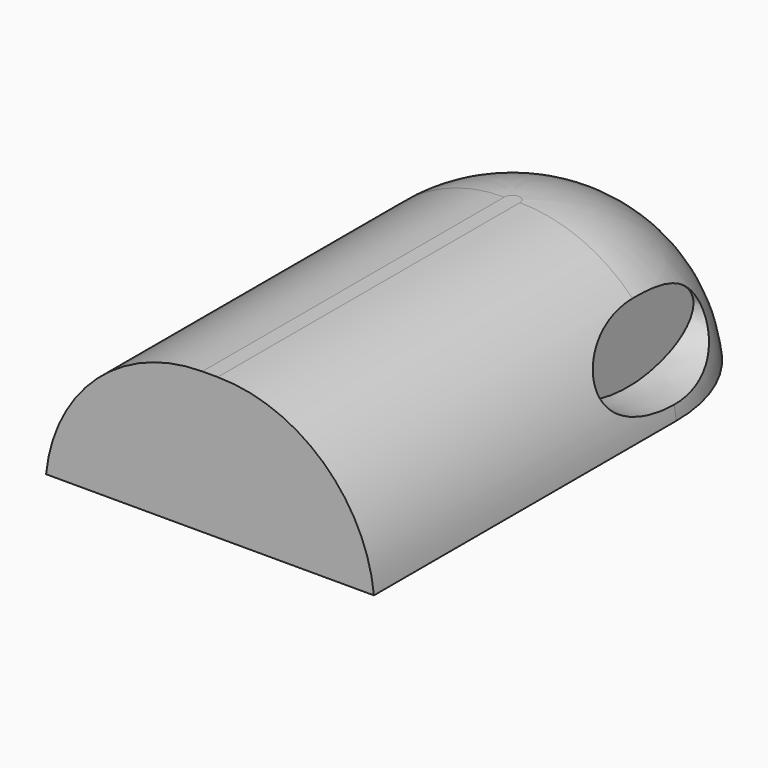
from build123d import *

# Parameters (mm, degrees)
F1_DEPTH    = 34.29
F2_T1_DEPTH = 186.4119082094
F2_T4_ANGLE = 180
F4_DEPTH    = 50.8
F6_DEPTH    = 27.94


# Not quite as in the source:
# - a fillet or chamfer that OpenCascade refuses, or shapes differently, is made with other operations: its cross-section is extruded or revolved along the edge and cut away or added


with BuildPart() as f1:
    # F0 (on Top) → F1 (new body)
    with BuildSketch(Plane.XY):
        with BuildLine():
            ThreePointArc((-39.772413671, 45.8196774125), (0, 6.0472637415), (39.772413671, 45.8196774125))
            Line((39.772413671, 45.8196774125), (-39.772413671, 45.8196774125))
        make_face()
        with BuildLine():
            Line((-39.772413671, 45.8196774125), (39.772413671, 45.8196774125))
            ThreePointArc((39.772413671, 45.8196774125), (0, 85.5920910835), (-39.772413671, 45.8196774125))
        make_face()
        with BuildLine():
            Line((39.772413671, -45.8196774125), (39.772413671, 45.8196774125))
            ThreePointArc((39.772413671, 45.8196774125), (0, 6.0472637415), (-39.772413671, 45.8196774125))
            Line((-39.772413671, 45.8196774125), (-39.772413671, -45.8196774125))
            Line((-39.772413671, -45.8196774125), (39.772413671, -45.8196774125))
        make_face()
    extrude(amount=F1_DEPTH)

    # F2: fillet of radius 38.1 on 3 edges, made by hand

    # F2_s2 → F2_t1 (cut)
    with BuildSketch(Plane.XZ.offset(-45.8196774125)):
        with BuildLine():
            ThreePointArc((-39.772413671, 0), (-27.4216493001, 24.4457162358), (-1.8633923173, 34.29))
            Line((-1.8633923173, 34.29), (-39.772413671, 34.29))
            Line((-39.772413671, 34.29), (-39.772413671, 0))
        make_face()
        with BuildLine():
            ThreePointArc((39.772413671, 0), (27.4216493001, 24.4457162358), (1.8633923173, 34.29))
            Line((1.8633923173, 34.29), (39.772413671, 34.29))
            Line((39.772413671, 34.29), (39.772413671, 0))
        make_face()
    extrude(amount=F2_T1_DEPTH, mode=Mode.SUBTRACT)

    # F2_s3 → F2_t4 (revolve, cut)
    with BuildSketch(Plane.XZ.offset(-45.8196774125)):
        with BuildLine():
            ThreePointArc((39.772413671, 0), (27.4216493001, 24.4457162358), (1.8633923173, 34.29))
            Line((1.8633923173, 34.29), (39.772413671, 34.29))
            Line((39.772413671, 34.29), (39.772413671, 0))
        make_face()
    revolve(axis=Axis((0, 45.8196774125, 34.29), (0, 0, 1)), revolution_arc=F2_T4_ANGLE, mode=Mode.SUBTRACT)

    # F3 (on Right) → F4 (cut)
    with BuildSketch(Plane.YZ):
        with BuildLine():
            add(Edge.make_bspline(
                [(26.3266563416, 13.0248842761), (26.3266563416, -3.7878693164), (55.981522426, 4.6185074799), (85.6363885105, 13.0248842761), (55.981522426, 21.4312610723), (26.3266563416, 29.8376378686), (26.3266563416, 13.0248842761)],
                knots=[0, 0, 0, 2.0943951024, 2.0943951024, 4.1887902048, 4.1887902048, 6.2831853072, 6.2831853072, 6.2831853072], degree=2, weights=[1, 0.5, 1, 0.5, 1, 0.5, 1]))
        make_face()
    extrude(amount=F4_DEPTH, mode=Mode.SUBTRACT)

    # F5 (on Right) → F6 (join)
    with BuildSketch(Plane.YZ):
        with BuildLine():
            add(Edge.make_bspline(
                [(65.8664852381, 13.2574718446), (65.8664852381, 30.580146327), (34.8160881549, 21.9188090858), (3.7656910717, 13.2574718446), (34.8160881549, 4.5961346033), (65.8664852381, -4.0652026379), (65.8664852381, 13.2574718446)],
                knots=[0, 0, 0, 2.0943951024, 2.0943951024, 4.1887902048, 4.1887902048, 6.2831853072, 6.2831853072, 6.2831853072], degree=2, weights=[1, 0.5, 1, 0.5, 1, 0.5, 1]))
        make_face()
    extrude(amount=F6_DEPTH)


solid = f1.part
